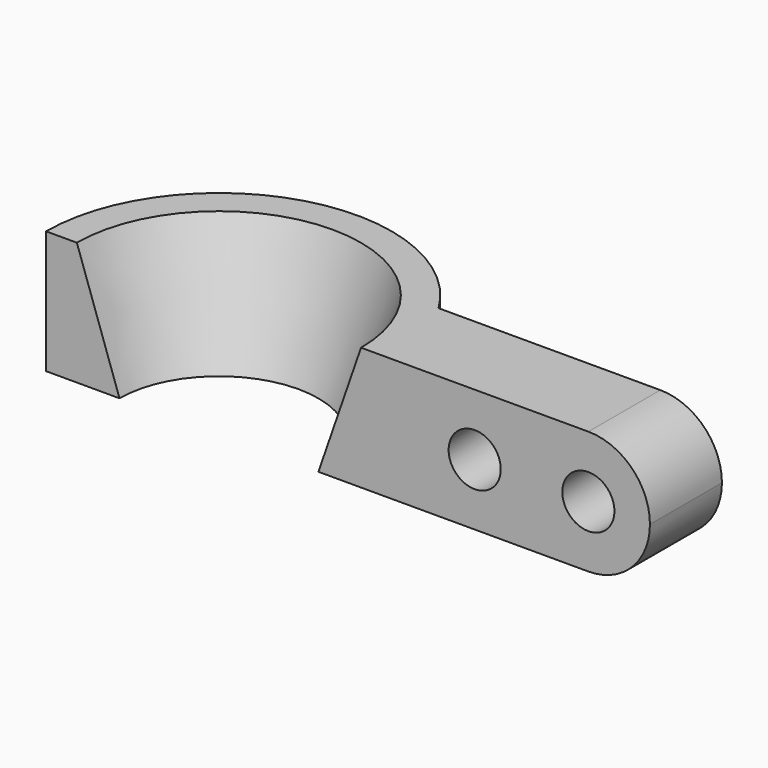
from build123d import *

# Parameters (mm, degrees)
F1_DEPTH = 52
F4_R     = 11
F5_DEPTH = 73.001
F6_R     = 25.99999


# Not quite as in the source:
# - a fillet or chamfer is up to 0.001 mm smaller than in the source, because OpenCascade refuses the exact size


with BuildPart() as f1:
    # F0 (on Top) → F1 (new body)
    with BuildSketch(Plane.XY):
        with BuildLine():
            Line((182, 38), (62.329768169, 38))
            ThreePointArc((62.329768169, 38), (-19.7348286497, 70.2818364741), (-73, 0))
            Line((-73, 0), (-60, 0))
            ThreePointArc((-60, 0), (0, 60), (60, 0))
            Line((60, 0), (182, 0))
            Line((182, 0), (182, 38))
        make_face()
        with BuildLine():
            ThreePointArc((60, 0), (0, 60), (-60, 0))
            Line((-60, 0), (-42, 0))
            ThreePointArc((-42, 0), (0, 42), (42, 0))
            Line((42, 0), (60, 0))
        make_face()
    extrude(amount=F1_DEPTH)

    # F2 (on face) → F3 (revolve, cut)
    with BuildSketch(Plane.XZ):
        Polygon((-60, 52), (-42, 0), (-42, 52), align=None)
    revolve(axis=Axis((0, 0, 26.0027386248), (0, 0, -1)), mode=Mode.SUBTRACT)

    # F4 (on face) → F5 (cut, through all)
    with BuildSketch(Plane.XZ):
        with Locations((108, 26)):
            Circle(F4_R)
        with Locations((156, 26)):
            Circle(F4_R)
    extrude(amount=-F5_DEPTH, mode=Mode.SUBTRACT)

    # F6 (radius 26 in the source; OpenCascade refuses exactly that, so slightly less here)
    f6_edges = [f1.edges().sort_by_distance(p)[0] for p in [
        (182, 19, 52),
        (182, 19, 0),
    ]]
    fillet(f6_edges, radius=F6_R)


solid = f1.part
